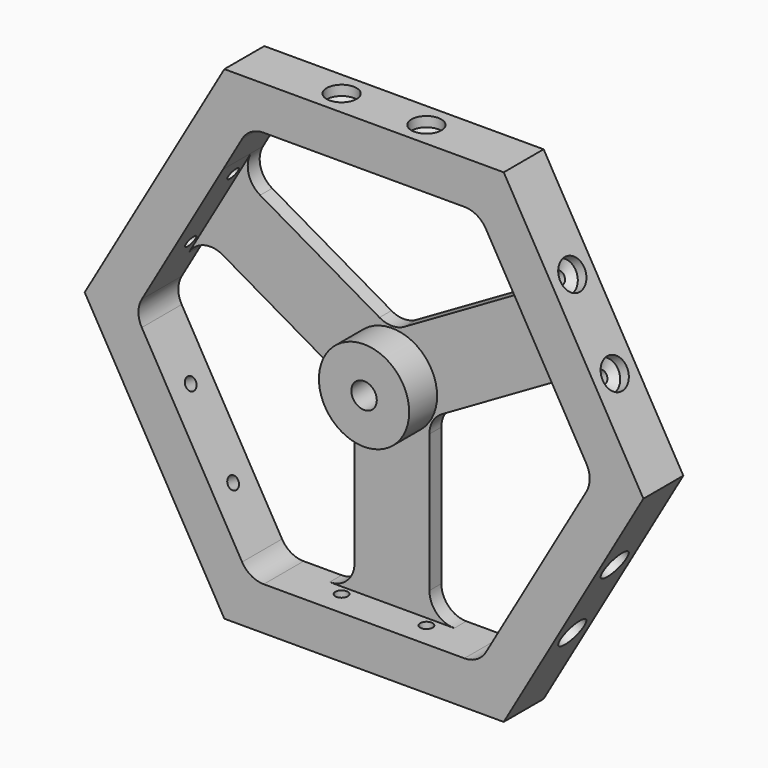
from build123d import *

# Parameters (mm, degrees)
F0_R      = 9.0451569713
F1_DEPTH  = 3
F2_DEPTH  = 10
F8_D      = 6
F8_DEPTH  = 2
F8_TIP    = 1.8025818571
F9_D      = 2.5
F9_DEPTH  = 13.5
F9_START  = 3.0515061
F9_TIP    = 0.7510757738
F10_D     = 2.5
F10_DEPTH = 13.5
F10_TIP   = 0.7510757738
F11_D     = 6
F11_DEPTH = 2
F11_TIP   = 1.8025818571
F12_D     = 6
F12_DEPTH = 2
F12_TIP   = 1.8025818571
F13_D     = 2.5
F13_DEPTH = 13.5
F13_START = 3.0515061
F13_TIP   = 0.7510757738
F15_D     = 2.5
F15_DEPTH = 13.5
F15_TIP   = 0.7510757738
F16_D     = 6
F16_DEPTH = 2
F16_TIP   = 1.8025818571
F17_D     = 6
F17_DEPTH = 2
F17_TIP   = 1.8025818571
F18_D     = 2.5
F18_DEPTH = 13.5
F18_START = 3.0515061
F18_TIP   = 0.7510757738
F19_D     = 2.5
F19_DEPTH = 13.5
F19_TIP   = 0.7510757738
F20_D     = 6
F20_DEPTH = 2
F20_TIP   = 1.8025818571
F21_D     = 5.1054
F21_DEPTH = 15.81
F21_TIP   = 1.5338169022


with BuildPart() as f1:
    # F0 (on Front) → F1 (new body)
    with BuildSketch(Plane.XZ):
        Polygon((28, -48.4974226119), (56, 0), (28, 48.4974226119), (-28, 48.4974226119), (-56, 0), (-28, -48.4974226119), align=None)
        with BuildLine():
            ThreePointArc((44.556624327, 2.5), (45.2264973081, 0), (44.556624327, -2.5))
            Line((44.556624327, -2.5), (24.443375673, -37.3371685741))
            ThreePointArc((24.443375673, -37.3371685741), (22.6132486541, -39.167295593), (20.1132486541, -39.8371685741))
            Line((20.1132486541, -39.8371685741), (12.5, -39.8371685741))
            Line((12.5, -39.8371685741), (-12.5, -39.8371685741))
            Line((-12.5, -39.8371685741), (-20.1132486541, -39.8371685741))
            ThreePointArc((-20.1132486541, -39.8371685741), (-22.6132486541, -39.167295593), (-24.443375673, -37.3371685741))
            Line((-24.443375673, -37.3371685741), (-44.556624327, -2.5))
            ThreePointArc((-44.556624327, -2.5), (-45.2264973081, 0), (-44.556624327, 2.5))
            Line((-44.556624327, 2.5), (-40.75, 9.0932667397))
            Line((-40.75, 9.0932667397), (-28.25, 30.7439018343))
            Line((-28.25, 30.7439018343), (-24.443375673, 37.3371685741))
            ThreePointArc((-24.443375673, 37.3371685741), (-22.6132486541, 39.167295593), (-20.1132486541, 39.8371685741))
            Line((-20.1132486541, 39.8371685741), (20.1132486541, 39.8371685741))
            ThreePointArc((20.1132486541, 39.8371685741), (22.6132486541, 39.167295593), (24.443375673, 37.3371685741))
            Line((24.443375673, 37.3371685741), (28.25, 30.7439018343))
            Line((28.25, 30.7439018343), (40.75, 9.0932667397))
            Line((40.75, 9.0932667397), (44.556624327, 2.5))
        make_face(mode=Mode.SUBTRACT)
        with BuildLine():
            ThreePointArc((33.9198729811, 10.9233937587), (37.7139682066, 11.4228958712), (40.75, 9.0932667397))
            Line((40.75, 9.0932667397), (28.25, 30.7439018343))
            ThreePointArc((28.25, 30.7439018343), (28.7495021125, 26.9498066088), (26.4198729811, 23.9137748154))
            Line((26.4198729811, 23.9137748154), (2.5, 10.1036297108))
            ThreePointArc((2.5, 10.1036297108), (0, 9.4337567297), (-2.5, 10.1036297108))
            Line((-2.5, 10.1036297108), (-26.4198729811, 23.9137748154))
            ThreePointArc((-26.4198729811, 23.9137748154), (-28.7495021125, 26.9498066088), (-28.25, 30.7439018343))
            Line((-28.25, 30.7439018343), (-40.75, 9.0932667397))
            ThreePointArc((-40.75, 9.0932667397), (-37.7139682066, 11.4228958712), (-33.9198729811, 10.9233937587))
            Line((-33.9198729811, 10.9233937587), (-10, -2.8867513459))
            ThreePointArc((-10, -2.8867513459), (-8.1698729811, -4.7168783649), (-7.5, -7.2168783649))
            Line((-7.5, -7.2168783649), (-7.5, -34.8371685741))
            ThreePointArc((-7.5, -34.8371685741), (-8.9644660941, -38.37270248), (-12.5, -39.8371685741))
            Line((-12.5, -39.8371685741), (12.5, -39.8371685741))
            ThreePointArc((12.5, -39.8371685741), (8.9644660941, -38.37270248), (7.5, -34.8371685741))
            Line((7.5, -34.8371685741), (7.5, -7.2168783649))
            ThreePointArc((7.5, -7.2168783649), (8.1698729811, -4.7168783649), (10, -2.8867513459))
            Line((10, -2.8867513459), (33.9198729811, 10.9233937587))
        make_face()
        Circle(F0_R, mode=Mode.SUBTRACT)
        Circle(F0_R)
    extrude(amount=F1_DEPTH)

    # F0 (on Front) → F2 (join)
    with BuildSketch(Plane.XZ):
        Polygon((28, -48.4974226119), (56, 0), (28, 48.4974226119), (-28, 48.4974226119), (-56, 0), (-28, -48.4974226119), align=None)
        with BuildLine():
            ThreePointArc((44.556624327, 2.5), (45.2264973081, 0), (44.556624327, -2.5))
            Line((44.556624327, -2.5), (24.443375673, -37.3371685741))
            ThreePointArc((24.443375673, -37.3371685741), (22.6132486541, -39.167295593), (20.1132486541, -39.8371685741))
            Line((20.1132486541, -39.8371685741), (12.5, -39.8371685741))
            Line((12.5, -39.8371685741), (-12.5, -39.8371685741))
            Line((-12.5, -39.8371685741), (-20.1132486541, -39.8371685741))
            ThreePointArc((-20.1132486541, -39.8371685741), (-22.6132486541, -39.167295593), (-24.443375673, -37.3371685741))
            Line((-24.443375673, -37.3371685741), (-44.556624327, -2.5))
            ThreePointArc((-44.556624327, -2.5), (-45.2264973081, 0), (-44.556624327, 2.5))
            Line((-44.556624327, 2.5), (-40.75, 9.0932667397))
            Line((-40.75, 9.0932667397), (-28.25, 30.7439018343))
            Line((-28.25, 30.7439018343), (-24.443375673, 37.3371685741))
            ThreePointArc((-24.443375673, 37.3371685741), (-22.6132486541, 39.167295593), (-20.1132486541, 39.8371685741))
            Line((-20.1132486541, 39.8371685741), (20.1132486541, 39.8371685741))
            ThreePointArc((20.1132486541, 39.8371685741), (22.6132486541, 39.167295593), (24.443375673, 37.3371685741))
            Line((24.443375673, 37.3371685741), (28.25, 30.7439018343))
            Line((28.25, 30.7439018343), (40.75, 9.0932667397))
            Line((40.75, 9.0932667397), (44.556624327, 2.5))
        make_face(mode=Mode.SUBTRACT)
        Circle(F0_R)
    extrude(amount=F2_DEPTH)

    # F8
    with Locations(Plane(origin=(0, 0, -48.4974226119), x_dir=(1, 0, 0), z_dir=(0, 0, -1))):
        with Locations((-8.5, 5), (8.5, 5)):
            Hole(F8_D / 2, depth=F8_DEPTH)
            with Locations((0, 0, -(F8_DEPTH + F8_TIP / 2))):  # 118° drill point
                Cone(0, F8_D / 2, F8_TIP, mode=Mode.SUBTRACT)

    # F9
    # its depths count from where the whole tool has entered the part; down to there all is cleared
    with Locations(Plane(origin=(0, 0, -48.4974226119), x_dir=(1, 0, 0), z_dir=(0, 0, -1)).offset(-F9_START)):
        with Locations((-8.5, 5), (8.5, 5)):
            Hole(F9_D / 2, depth=F9_DEPTH)
            with Locations((0, 0, -(F9_DEPTH + F9_TIP / 2))):  # 118° drill point
                Cone(0, F9_D / 2, F9_TIP, mode=Mode.SUBTRACT)

    # F10
    with Locations(Plane(origin=(42, 0, -24.248711306), x_dir=(0, 1, 0), z_dir=(0.8660254038, 0, -0.5))):
        with Locations((-5, -8.5), (-5, 8.5)):
            Hole(F10_D / 2, depth=F10_DEPTH)
            with Locations((0, 0, -(F10_DEPTH + F10_TIP / 2))):  # 118° drill point
                Cone(0, F10_D / 2, F10_TIP, mode=Mode.SUBTRACT)

    # F11
    with Locations(Plane(origin=(42, 0, -24.248711306), x_dir=(0, 1, 0), z_dir=(0.8660254038, 0, -0.5))):
        with Locations((-5, -8.5), (-5, 8.5)):
            Hole(F11_D / 2, depth=F11_DEPTH)
            with Locations((0, 0, -(F11_DEPTH + F11_TIP / 2))):  # 118° drill point
                Cone(0, F11_D / 2, F11_TIP, mode=Mode.SUBTRACT)

    # F12
    with Locations(Plane(origin=(42, 0, 24.248711306), x_dir=(0, 1, 0), z_dir=(0.8660254038, 0, 0.5))):
        with Locations((-5, -8.5), (-5, 8.5)):
            Hole(F12_D / 2, depth=F12_DEPTH)
            with Locations((0, 0, -(F12_DEPTH + F12_TIP / 2))):  # 118° drill point
                Cone(0, F12_D / 2, F12_TIP, mode=Mode.SUBTRACT)

    # F13
    # its depths count from where the whole tool has entered the part; down to there all is cleared
    with Locations(Plane(origin=(42, 0, 24.248711306), x_dir=(0, 1, 0), z_dir=(0.8660254038, 0, 0.5)).offset(-F13_START)):
        with Locations((-5, -8.5), (-5, 8.5)):
            Hole(F13_D / 2, depth=F13_DEPTH)
            with Locations((0, 0, -(F13_DEPTH + F13_TIP / 2))):  # 118° drill point
                Cone(0, F13_D / 2, F13_TIP, mode=Mode.SUBTRACT)

    # F15
    with Locations(Plane.XY.offset(48.4974226119)):
        with Locations((8.5, -5), (-8.5, -5)):
            Hole(F15_D / 2, depth=F15_DEPTH)
            with Locations((0, 0, -(F15_DEPTH + F15_TIP / 2))):  # 118° drill point
                Cone(0, F15_D / 2, F15_TIP, mode=Mode.SUBTRACT)

    # F16
    with Locations(Plane.XY.offset(48.4974226119)):
        with Locations((8.5, -5), (-8.5, -5)):
            Hole(F16_D / 2, depth=F16_DEPTH)
            with Locations((0, 0, -(F16_DEPTH + F16_TIP / 2))):  # 118° drill point
                Cone(0, F16_D / 2, F16_TIP, mode=Mode.SUBTRACT)

    # F17
    with Locations(Plane(origin=(-42, 0, 24.248711306), x_dir=(0, -1, 0), z_dir=(-0.8660254038, 0, 0.5))):
        with Locations((5, 8.5), (5, -8.5)):
            Hole(F17_D / 2, depth=F17_DEPTH)
            with Locations((0, 0, -(F17_DEPTH + F17_TIP / 2))):  # 118° drill point
                Cone(0, F17_D / 2, F17_TIP, mode=Mode.SUBTRACT)

    # F18
    # its depths count from where the whole tool has entered the part; down to there all is cleared
    with Locations(Plane(origin=(-42, 0, 24.248711306), x_dir=(0, -1, 0), z_dir=(-0.8660254038, 0, 0.5)).offset(-F18_START)):
        with Locations((5, 8.5), (5, -8.5)):
            Hole(F18_D / 2, depth=F18_DEPTH)
            with Locations((0, 0, -(F18_DEPTH + F18_TIP / 2))):  # 118° drill point
                Cone(0, F18_D / 2, F18_TIP, mode=Mode.SUBTRACT)

    # F19
    with Locations(Plane(origin=(-42, 0, -24.248711306), x_dir=(0, -1, 0), z_dir=(-0.8660254038, 0, -0.5))):
        with Locations((5, 8.5), (5, -8.5)):
            Hole(F19_D / 2, depth=F19_DEPTH)
            with Locations((0, 0, -(F19_DEPTH + F19_TIP / 2))):  # 118° drill point
                Cone(0, F19_D / 2, F19_TIP, mode=Mode.SUBTRACT)

    # F20
    with Locations(Plane(origin=(-42, 0, -24.248711306), x_dir=(0, -1, 0), z_dir=(-0.8660254038, 0, -0.5))):
        with Locations((5, 8.5), (5, -8.5)):
            Hole(F20_D / 2, depth=F20_DEPTH)
            with Locations((0, 0, -(F20_DEPTH + F20_TIP / 2))):  # 118° drill point
                Cone(0, F20_D / 2, F20_TIP, mode=Mode.SUBTRACT)

    # F21
    with Locations(Plane(origin=(0, 0, 0), x_dir=(1, 0, 0), z_dir=(0, 1, 0))):
        with Locations((0, 0)):
            Hole(F21_D / 2, depth=F21_DEPTH)
            with Locations((0, 0, -(F21_DEPTH + F21_TIP / 2))):  # 118° drill point
                Cone(0, F21_D / 2, F21_TIP, mode=Mode.SUBTRACT)


solid = f1.part
